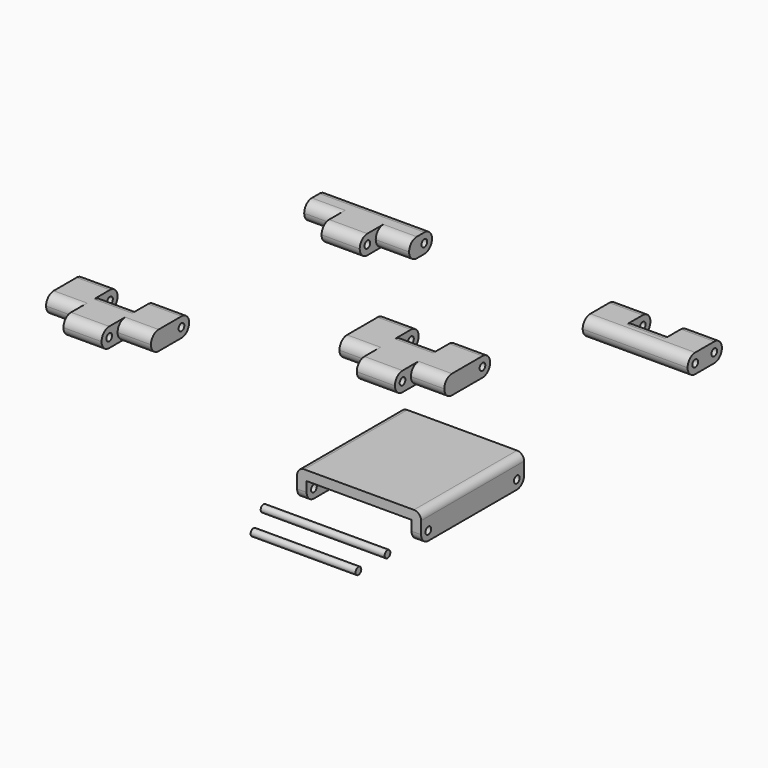
from build123d import *

# Parameters (mm, degrees)
F1_DEPTH  = 4
F2_R      = 1.99999
F2_2_R    = 1.99999
F2_3_R    = 1.99999
F2_4_R    = 1.99999
F3_R      = 0.75
F4_DEPTH  = 22
F5_R      = 0.75
F6_DEPTH  = 10
F7_R      = 0.75
F8_DEPTH  = 22
F9_R      = 0.75
F10_DEPTH = 22
F11_R     = 0.75
F12_DEPTH = 10
F13_R     = 0.75
F14_DEPTH = 22
F15_R     = 0.75
F16_DEPTH = 10
F0_W      = 2
F0_H      = 27
F0_W_2    = 22
F17_DEPTH = 6
F18_DEPTH = 4
F19_R     = 1.9
F20_R     = 0.75
F21_DEPTH = 26
F22_DEPTH = 26
F23_DEPTH = 22
F24_R     = 1.5


# Not quite as in the source:
# - a fillet or chamfer is up to 0.001 mm smaller than in the source, because OpenCascade refuses the exact size


with BuildPart() as f1:
    # F0 (on Top) → F1 (new body)
    with BuildSketch(Plane.XY):
        Polygon((-38.8388755443, 34.7694223676), (-45.8388755443, 34.7694223676), (-45.8388755443, 28.7694223676), (-38.8388755443, 28.7694223676), (-38.8388755443, 24.5694223676), (-34.8388755443, 24.5694223676), (-30.8388755443, 24.5694223676), (-30.8388755443, 28.7694223676), (-23.8388755443, 28.7694223676), (-23.8388755443, 34.7694223676), (-30.8388755443, 34.7694223676), align=None)
    extrude(amount=F1_DEPTH)

    # F2 (radius 2 in the source; OpenCascade refuses exactly that, so slightly less here)
    f2_edges = [f1.edges().sort_by_distance(p)[0] for p in [
        (-34.838876, 34.769422, 4),
        (-42.338876, 28.769422, 4),
        (-42.338876, 28.769422, 0),
        (-27.338876, 28.769422, 4),
        (-27.338876, 28.769422, 0),
        (-34.838876, 34.769422, 0),
        (-34.838876, 24.569422, 0),
        (-34.838876, 24.569422, 4),
    ]]
    fillet(f2_edges, radius=F2_R)

    # F3 (on face) → F4 (cut)
    with BuildSketch(Plane(origin=(-45.8388755443, 0, 0), x_dir=(0, -1, 0), z_dir=(-1, 0, 0))):
        with Locations((-32.7694223676, 2)):
            Circle(F3_R)
    extrude(amount=-F4_DEPTH, mode=Mode.SUBTRACT)

    # F5 (on face) → F6 (cut)
    with BuildSketch(Plane(origin=(-38.8388755443, 0, 0), x_dir=(0, -1, 0), z_dir=(-1, 0, 0))):
        with Locations((-26.5694223676, 2)):
            Circle(F5_R)
    extrude(amount=-F6_DEPTH, mode=Mode.SUBTRACT)


with BuildPart() as f1b:
    # F0 (on Top) → F1, piece 2 (new body)
    with BuildSketch(Plane.XY):
        Polygon((22.4313167212, 34.190556467), (15.4313167212, 34.190556467), (15.4313167212, 25.190556467), (22.4313167212, 25.190556467), (30.4313167212, 25.190556467), (37.4313167212, 25.190556467), (37.4313167212, 34.190556467), (30.4313167212, 34.190556467), (30.4313167212, 29.990556467), (26.4313167212, 29.990556467), (22.4313167212, 29.990556467), align=None)
    extrude(amount=F1_DEPTH)

    # F2#2 (radius 2 in the source; OpenCascade refuses exactly that, so slightly less here)
    f2_2_edges = [f1b.edges().sort_by_distance(p)[0] for p in [
        (18.931317, 34.190556, 4),
        (33.931317, 34.190556, 4),
        (26.431317, 25.190556, 4),
        (26.431317, 25.190556, 0),
        (18.931317, 34.190556, 0),
        (33.931317, 34.190556, 0),
        (26.431317, 29.990556, 0),
        (26.431317, 29.990556, 4),
    ]]
    fillet(f2_2_edges, radius=F2_2_R)

    # F7 (on face) → F8 (cut)
    with BuildSketch(Plane(origin=(15.4313167212, 0, 0), x_dir=(0, -1, 0), z_dir=(-1, 0, 0))):
        with Locations((-32.190556467, 2)):
            Circle(F7_R)
        with Locations((-27.190556467, 2)):
            Circle(F7_R)
    extrude(amount=-F8_DEPTH, mode=Mode.SUBTRACT)


with BuildPart() as f1c:
    # F0 (on Top) → F1, piece 3 (new body)
    with BuildSketch(Plane.XY):
        Polygon((-4, 6.45), (-11, 6.45), (-11, -5.55), (-4, -5.55), (-4, -9.75), (0, -9.75), (4, -9.75), (4, -5.55), (11, -5.55), (11, 6.45), (4, 6.45), (4, 2.25), (0, 2.25), (-4, 2.25), align=None)
    extrude(amount=F1_DEPTH)

    # F2#3 (radius 2 in the source; OpenCascade refuses exactly that, so slightly less here)
    f2_3_edges = [f1c.edges().sort_by_distance(p)[0] for p in [
        (-7.5, 6.45, 4),
        (7.5, 6.45, 4),
        (7.5, -5.55, 4),
        (-7.5, -5.55, 4),
        (7.5, 6.45, 0),
        (-7.5, 6.45, 0),
        (-7.5, -5.55, 0),
        (7.5, -5.55, 0),
        (0, 2.25, 0),
        (0, -9.75, 0),
        (0, 2.25, 4),
        (0, -9.75, 4),
    ]]
    fillet(f2_3_edges, radius=F2_3_R)

    # F9 (on face) → F10 (cut)
    with BuildSketch(Plane(origin=(-11, 0, 0), x_dir=(0, -1, 0), z_dir=(-1, 0, 0))):
        with Locations((-4.45, 2)):
            Circle(F9_R)
    extrude(amount=-F10_DEPTH, mode=Mode.SUBTRACT)

    # F11 (on face) → F12 (cut)
    with BuildSketch(Plane(origin=(-4, 0, 0), x_dir=(0, -1, 0), z_dir=(-1, 0, 0))):
        with Locations((7.75, 2)):
            Circle(F11_R)
    extrude(amount=-F12_DEPTH, mode=Mode.SUBTRACT)


with BuildPart() as f1d:
    # F0 (on Top) → F1, piece 4 (new body)
    with BuildSketch(Plane.XY):
        Polygon((-51.2933294001, -13.3388710316), (-58.2933294001, -13.3388710316), (-58.2933294001, -23.3388710316), (-51.2933294001, -23.3388710316), (-51.2933294001, -27.5388710316), (-47.2933294001, -27.5388710316), (-43.2933294001, -27.5388710316), (-43.2933294001, -23.3388710316), (-36.2933294001, -23.3388710316), (-36.2933294001, -13.3388710316), (-43.2933294001, -13.3388710316), (-43.2933294001, -17.5388710316), (-47.2933294001, -17.5388710316), (-51.2933294001, -17.5388710316), align=None)
    extrude(amount=F1_DEPTH)

    # F2#4 (radius 2 in the source; OpenCascade refuses exactly that, so slightly less here)
    f2_4_edges = [f1d.edges().sort_by_distance(p)[0] for p in [
        (-54.793329, -13.338871, 4),
        (-39.793329, -13.338871, 4),
        (-54.793329, -23.338871, 4),
        (-39.793329, -23.338871, 4),
        (-54.793329, -13.338871, 0),
        (-39.793329, -13.338871, 0),
        (-39.793329, -23.338871, 0),
        (-54.793329, -23.338871, 0),
        (-47.293329, -27.538871, 0),
        (-47.293329, -17.538871, 0),
        (-47.293329, -27.538871, 4),
        (-47.293329, -17.538871, 4),
    ]]
    fillet(f2_4_edges, radius=F2_4_R)

    # F13 (on face) → F14 (cut)
    with BuildSketch(Plane(origin=(-58.2933294001, 0, 0), x_dir=(0, -1, 0), z_dir=(-1, 0, 0))):
        with Locations((15.3388710316, 2)):
            Circle(F13_R)
    extrude(amount=-F14_DEPTH, mode=Mode.SUBTRACT)

    # F15 (on face) → F16 (cut)
    with BuildSketch(Plane(origin=(-51.2933294001, 0, 0), x_dir=(0, -1, 0), z_dir=(-1, 0, 0))):
        with Locations((25.5388710316, 2)):
            Circle(F15_R)
    extrude(amount=-F16_DEPTH, mode=Mode.SUBTRACT)


with BuildPart() as f17:
    # F0 (on Top) → F17 (new body)
    with BuildSketch(Plane.XY):
        with Locations((15.223434031, -34.6688529253)):
            Rectangle(F0_W, F0_H)
        with Locations((27.223434031, -34.6688529253)):
            Rectangle(F0_W_2, F0_H)
        with Locations((39.223434031, -34.6688529253)):
            Rectangle(F0_W, F0_H)
    extrude(amount=F17_DEPTH)

    # F0 (on Top) → F18 (cut)
    with BuildSketch(Plane.XY):
        with Locations((27.223434031, -34.6688529253)):
            Rectangle(F0_W_2, F0_H)
    extrude(amount=F18_DEPTH, mode=Mode.SUBTRACT)

    # F19
    f19_edges = [f17.edges().sort_by_distance(p)[0] for p in [
        (39.223434, -48.168853, 0),
        (39.223434, -21.168853, 0),
        (15.223434, -48.168853, 0),
        (15.223434, -21.168853, 0),
    ]]
    fillet(f19_edges, radius=F19_R)

    # F20 (on face) → F21 (cut)
    with BuildSketch(Plane.YZ.offset(40.223434031)):
        with Locations((-46.2688529253, 1.9)):
            Circle(F20_R)
        with Locations((-23.0688529253, 1.9)):
            Circle(F20_R)
    extrude(amount=-F21_DEPTH, mode=Mode.SUBTRACT)

    # F24
    f24_edges = [f17.edges().sort_by_distance(p)[0] for p in [
        (40.223434, -34.668853, 6),
        (14.223434, -34.668853, 6),
    ]]
    fillet(f24_edges, radius=F24_R)


with BuildPart() as f22:
    # F20 (on face) → F22 (new body)
    with BuildSketch(Plane.YZ.offset(40.223434031)):
        with Locations((-56.9708310068, 1.9)):
            Circle(F20_R)
    extrude(amount=-F22_DEPTH)


with BuildPart() as f23:
    # F20 (on face) → F23 (new body)
    with BuildSketch(Plane.YZ.offset(40.223434031)):
        with Locations((-64.6062120795, 1.9)):
            Circle(F20_R)
    extrude(amount=-F23_DEPTH)


solid = Compound([f1.part, f1b.part, f1c.part, f1d.part, f17.part, f22.part, f23.part])
